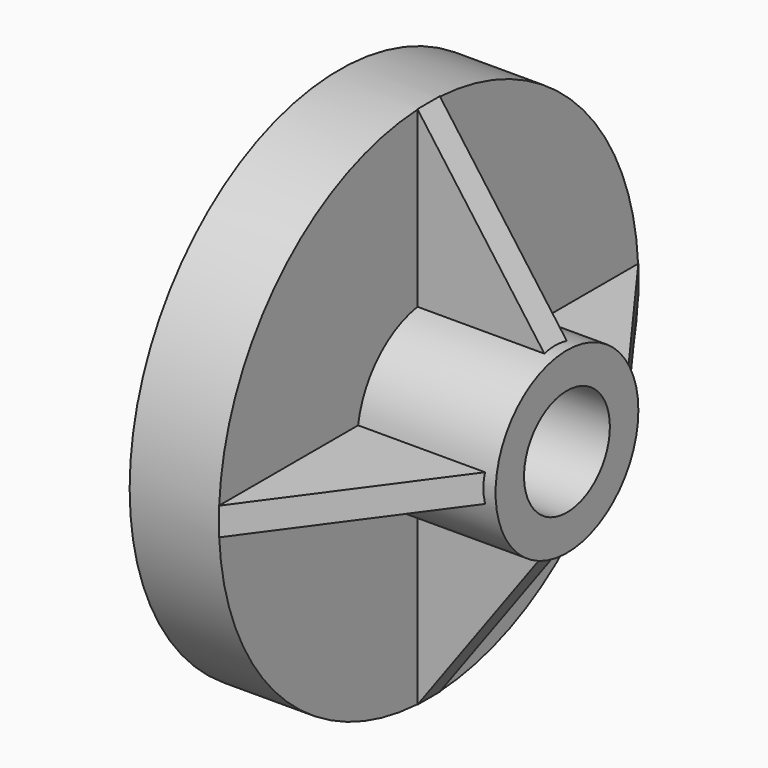
from build123d import *

# Parameters (mm, degrees)
F2_R            = 3.0529538636
F3_DEPTH        = 15.875
F5_DEPTH        = 0.79375
F5_DEPTH_BACK   = 0.79375
F5_COPIES_COUNT = 4
F6_R            = 3.175
F7_DEPTH        = 2.921


# Not quite as in the source:
# - a pattern or mirror of a feature is missing from the dataset's text; its kind, count and spacing are read off the source's solid


with BuildPart() as f1:
    # F0 (on Top) → F1 (revolve)
    with BuildSketch(Plane.XY):
        Polygon((0, 3.175), (0, 0), (15.875, 0), (15.875, 5.08), (8.001, 5.08), (8.001, 14.9225), (2.921, 14.9225), (2.921, 3.175), align=None)
    revolve(axis=Axis((7.9375, 0, 0), (-1, 0, 0)))

    # F2 (on face) → F3 (cut, through all)
    with BuildSketch(Plane.YZ.offset(15.875)):
        Circle(F2_R)
    extrude(amount=-F3_DEPTH, mode=Mode.SUBTRACT)

    # F4 (on Front) → F5 (join, two sides)
    with BuildSketch(Plane.XZ) as f5_sk:
        Polygon((15.875, 4.1275), (8.001, 14.9225), (8.001, 4.1275), align=None)
    f5 = extrude(amount=F5_DEPTH) + extrude(f5_sk.sketch, amount=-F5_DEPTH_BACK)

    # F5_copies: F5 ×4 about axis
    f5_copies_axis = Axis((0, 0, 0), (1, 0, 0))
    for i in range(1, F5_COPIES_COUNT):
        add(f5.rotate(f5_copies_axis, i * 360 / F5_COPIES_COUNT))

    # F6 (on face) → F7 (cut, through all)
    with BuildSketch(Plane(origin=(0, 0, 0), x_dir=(0, -1, 0), z_dir=(-1, 0, 0))):
        Circle(F6_R)
    extrude(amount=-F7_DEPTH, mode=Mode.SUBTRACT)


solid = f1.part
